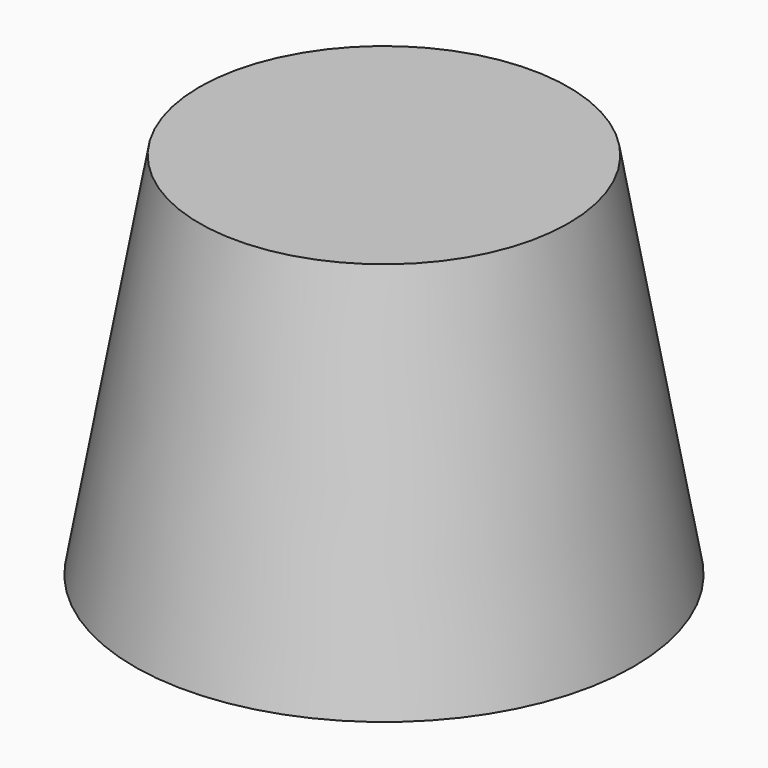
from build123d import *

# Parameters (mm, degrees)
F0_R     = 19.05
F1_DEPTH = 38.1
F1_TAPER = -10


with BuildPart() as f1:
    # F0 (on Top) → F1 (new body)
    with BuildSketch(Plane.XY):
        Circle(F0_R)
    extrude(amount=-F1_DEPTH, taper=F1_TAPER)


solid = f1.part
